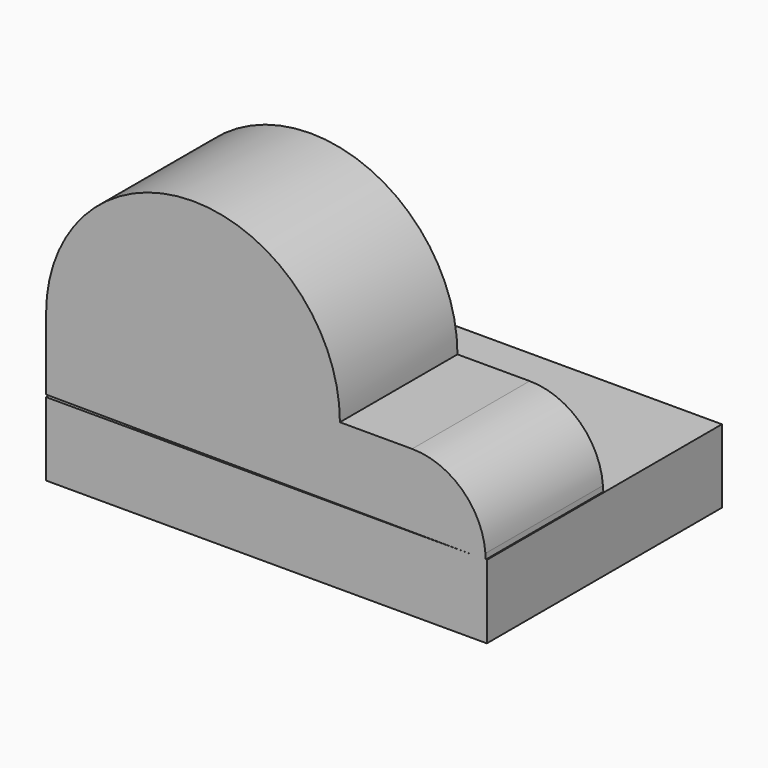
from build123d import *

# Parameters (mm, degrees)
F0_W     = 60
F0_H     = 40
F1_DEPTH = 10
F5_DEPTH = 20


# Not quite as in the source:
# - a feature of the source that left no trace in its solid (it failed there, or was rolled back) is left out


with BuildPart() as f1:
    # F0 (on Top) → F1 (new body)
    with BuildSketch(Plane.XY):
        with Locations((30, 20)):
            Rectangle(F0_W, F0_H)
    extrude(amount=F1_DEPTH)

    # F2 (on Front) → F5 (join)
    with BuildSketch(Plane.XZ):
        with BuildLine():
            Line((49.8285376106, 20), (40, 20))
            ThreePointArc((40, 20), (20, 40), (0, 20))
            Line((0, 20), (0, 10.3115513921))
            Line((0, 10.3115513921), (59.8550215364, 9.9916663021))
            Line((59.8550215364, 9.9916663021), (59.8027205061, 10.7181055402))
            ThreePointArc((59.8027205061, 10.7181055402), (56.6409874121, 17.3205551498), (49.8285376106, 20))
        make_face()
    extrude(amount=-F5_DEPTH)


solid = f1.part
